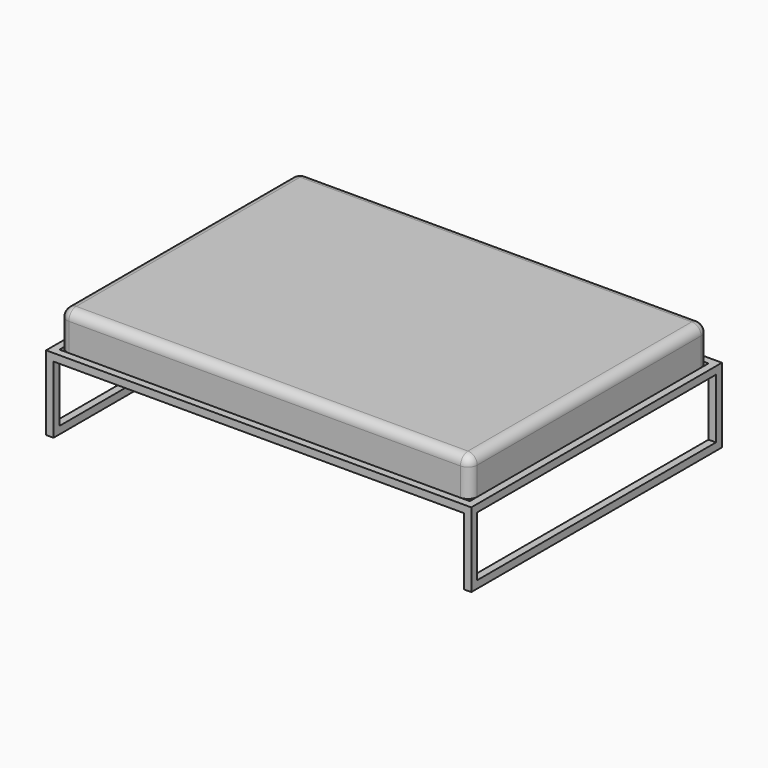
from build123d import *

# Parameters (mm, degrees)
F0_W     = 2280
F0_H     = 1680
F0_W_2   = 2200
F0_H_2   = 1600
F1_DEPTH = 400
F2_W     = 2200
F2_H     = 360
F3_DEPTH = 1680.001
F4_W     = 1600
F4_H     = 320
F5_DEPTH = 2280.001
F7_DEPTH = 200
F8_R     = 50


# Not quite as in the source:
# - the program builds the solid bodies; features that only make, move or delete a surface that nothing else refers to are left out


with BuildPart() as f1:
    # F0 (on Top) → F1 (new body)
    with BuildSketch(Plane.XY):
        Rectangle(F0_W, F0_H)
        Rectangle(F0_W_2, F0_H_2, mode=Mode.SUBTRACT)
    extrude(amount=-F1_DEPTH)

    # F2 (on face) → F3 (cut, through all)
    with BuildSketch(Plane.XZ.offset(840)):
        with Locations((0, -220)):
            Rectangle(F2_W, F2_H)
    extrude(amount=-F3_DEPTH, mode=Mode.SUBTRACT)

    # F4 (on face) → F5 (cut, through all)
    with BuildSketch(Plane(origin=(-1140, 0, 0), x_dir=(0, -1, 0), z_dir=(-1, 0, 0))):
        with Locations((0, -200)):
            Rectangle(F4_W, F4_H)
    extrude(amount=-F5_DEPTH, mode=Mode.SUBTRACT)


with BuildPart() as f7:
    # F0 (on Top) → F7 (new body)
    with BuildSketch(Plane.XY):
        Rectangle(F0_W_2, F0_H_2)
    extrude(amount=F7_DEPTH)

    # F8
    f8_edges = [f7.edges().sort_by_distance(p)[0] for p in [
        (-1100, 0, 200),
        (0, -800, 200),
        (-1100, -800, 100),
        (1100, -800, 100),
        (1100, 0, 200),
        (0, 800, 200),
        (1100, 800, 100),
        (-1100, 800, 100),
    ]]
    fillet(f8_edges, radius=F8_R)


solid = Compound([f1.part, f7.part])
